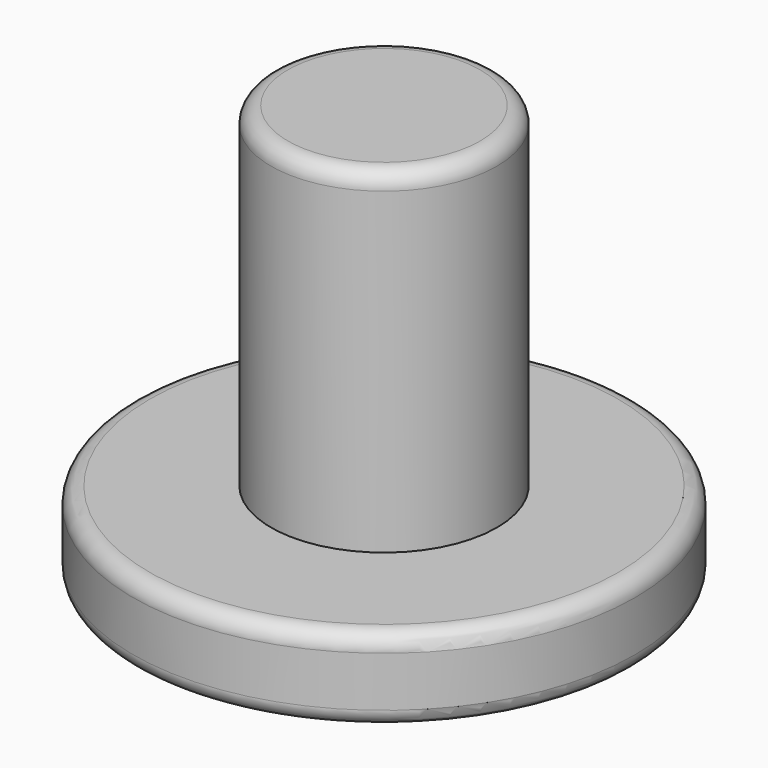
from build123d import *

# Parameters (mm, degrees)
F0_R     = 6.75
F1_DEPTH = 25
F0_R_2   = 15
F2_DEPTH = 5
F3_R     = 1


with BuildPart() as f1:
    # F0 (on Top) → F1 (new body)
    with BuildSketch(Plane.XY):
        Circle(F0_R)
    extrude(amount=F1_DEPTH)

    # F0 (on Top) → F2 (join)
    with BuildSketch(Plane.XY):
        Circle(F0_R_2)
        Circle(F0_R, mode=Mode.SUBTRACT)
    extrude(amount=F2_DEPTH)

    # F3
    f3_edges = [f1.edges().sort_by_distance(p)[0] for p in [
        (-15, 0, 0),
        (-15, 0, 5),
        (-6.75, 0, 25),
    ]]
    fillet(f3_edges, radius=F3_R)


solid = f1.part
